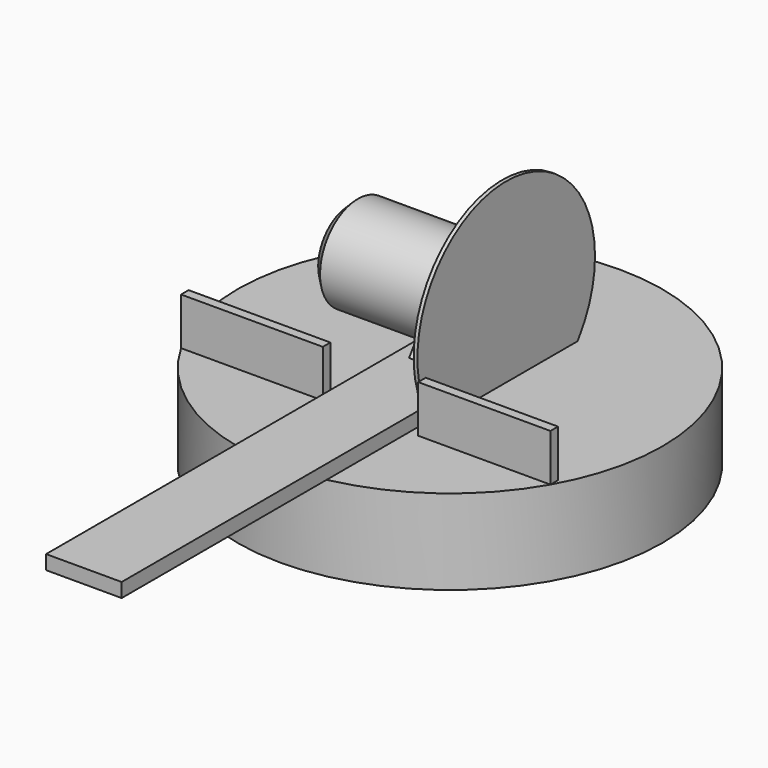
from build123d import *

# Parameters (mm, degrees)
F0_W          = 80
F0_H          = 600
F1_DEPTH      = 15
F3_DEPTH      = 43
F3_DEPTH_BACK = 120
F4_DEPTH      = 25
F4_DEPTH_BACK = 25
F5_R          = 117.5
F6_DEPTH      = 4
F8_W          = 25
F8_H          = 90
F10_R         = 30
F11_SIZE      = 10
F13_DEPTH     = 72.001
F14_T1_DEPTH  = 30
F14_T4_ANGLE  = 90
F14_T8_DEPTH  = 72.5
F14_S9_R      = 50
F14_T10_DEPTH = 38
F14_T14_DEPTH = 72.5
F14_S15_R     = 50
F14_T16_DEPTH = 38
F14_T18_ANGLE = 90
F14_T22_DEPTH = 67.4896230895
F14_T25_ANGLE = 180
F14_T27_ANGLE = 180
F14_T29_ANGLE = 90
F14_T31_ANGLE = 90
F14_T35_DEPTH = 67.4896230895
F14_T38_ANGLE = 180
F14_T40_ANGLE = 180
F15_R         = 225
F16_DEPTH     = 90
F17_W         = 140
F17_H         = 10
F17_W_2       = 150
F18_DEPTH     = 50


# Not quite as in the source:
# - a fillet or chamfer that OpenCascade refuses, or shapes differently, is made with other operations: its cross-section is extruded or revolved along the edge and cut away or added


with BuildPart() as f1:
    # F0 (on Top) → F1 (new body)
    with BuildSketch(Plane.XY):
        with Locations((0, -200)):
            Rectangle(F0_W, F0_H)
    extrude(amount=-F1_DEPTH)


with BuildPart() as f3:
    # F2 (on Right) → F3 (new body, two sides)
    with BuildSketch(Plane.YZ) as f3_sk:
        with BuildLine():
            Line((0, 55), (-28.6788218176, 14.0423977856))
            ThreePointArc((-28.6788218176, 14.0423977855), (0, 5), (28.6788218176, 14.0423977855))
            Line((28.6788218176, 14.0423977856), (0, 55))
        make_face()
        with BuildLine():
            ThreePointArc((28.6788218176, 14.0423977855), (44.3505416589, 31.9125693382), (50, 55))
            ThreePointArc((50, 55), (-23.0874306618, 99.3505416589), (-28.6788218176, 14.0423977855))
            Line((-28.6788218176, 14.0423977856), (0, 55))
            Line((0, 55), (28.6788218176, 14.0423977856))
        make_face()
    extrude(amount=F3_DEPTH)
    extrude(f3_sk.sketch, amount=-F3_DEPTH_BACK)

    # F2 (on Right) → F4 (join, two sides)
    with BuildSketch(Plane.YZ) as f4_sk:
        with BuildLine():
            ThreePointArc((28.6788218176, 14.0423977855), (0, 5), (-28.6788218176, 14.0423977855))
            Line((-28.6788218176, 14.0423977856), (-49.0145276747, -15))
            Line((-49.0145276747, -15), (49.0145276747, -15))
            Line((49.0145276747, -15), (28.6788218176, 14.0423977856))
        make_face()
    extrude(amount=F4_DEPTH)
    extrude(f4_sk.sketch, amount=-F4_DEPTH_BACK)

    # F8 (on offset) → F9 (join, up to the next surface of F3)
    with BuildSketch(Plane.XZ.offset(-120)):
        with Locations((-12.5, 50)):
            Rectangle(F8_W, F8_H)
    extrude(until=Until.NEXT)

    # F10
    f10_edges = [f3.edges().sort_by_distance(p)[0] for p in [
        (-12.5, 120, 95),
        (-12.5, 120, 5),
    ]]
    fillet(f10_edges, radius=F10_R)

    # F11
    f11_edges = [f3.edges().sort_by_distance(p)[0] for p in [
        (-120, 28.678822, 95.957602),
    ]]
    chamfer(f11_edges, length=F11_SIZE)

    # F12 (on face) → F13 (cut, through all)
    with BuildSketch(Plane(origin=(-25, 0, 0), x_dir=(0, -1, 0), z_dir=(-1, 0, 0))):
        with BuildLine():
            Line((-75, 35), (-75, 65))
            ThreePointArc((-75, 65), (-90, 80), (-105, 65))
            Line((-105, 65), (-105, 35))
            ThreePointArc((-105, 35), (-90, 20), (-75, 35))
        make_face()
    extrude(amount=-F13_DEPTH, mode=Mode.SUBTRACT)

    # F14: fillet of radius 5 on 18 edges, made by hand

    # F14_s2 → F14_t1 (cut)
    with BuildSketch(Plane.XY.offset(35)):
        with BuildLine():
            ThreePointArc((-25, 110), (-23.5355339059, 106.4644660941), (-20, 105))
            Line((-20, 105), (-25, 105))
            Line((-25, 105), (-25, 110))
        make_face()
        with BuildLine():
            ThreePointArc((0, 115), (-1.4644660941, 118.5355339059), (-5, 120))
            Line((-5, 120), (0, 120))
            Line((0, 120), (0, 115))
        make_face()
        with BuildLine():
            ThreePointArc((0, 110), (-1.4644660941, 106.4644660941), (-5, 105))
            Line((-5, 105), (0, 105))
            Line((0, 105), (0, 110))
        make_face()
        with BuildLine():
            ThreePointArc((-25, 115), (-23.5355339059, 118.5355339059), (-20, 120))
            Line((-20, 120), (-25, 120))
            Line((-25, 120), (-25, 115))
        make_face()
        with BuildLine():
            ThreePointArc((-25, 70), (-23.5355339059, 73.5355339059), (-20, 75))
            Line((-20, 75), (-25, 75))
            Line((-25, 75), (-25, 70))
        make_face()
        with BuildLine():
            ThreePointArc((0, 70), (-1.4644660941, 73.5355339059), (-5, 75))
            Line((-5, 75), (0, 75))
            Line((0, 75), (0, 70))
        make_face()
    extrude(amount=F14_T1_DEPTH, mode=Mode.SUBTRACT)

    # F14_s3 → F14_t4 (revolve, cut)
    with BuildSketch(Plane.XY.offset(65)):
        with BuildLine():
            ThreePointArc((-25, 115), (-23.5355339059, 118.5355339059), (-20, 120))
            Line((-20, 120), (-25, 120))
            Line((-25, 120), (-25, 115))
        make_face()
    revolve(axis=Axis((-25, 90, 65), (1, 0, 0)), revolution_arc=F14_T4_ANGLE, mode=Mode.SUBTRACT)


with BuildPart() as f6:
    # F5 (on face) → F6 (new body)
    with BuildSketch(Plane.YZ.offset(43)):
        with Locations((0, 55)):
            Circle(F5_R)
    extrude(amount=F6_DEPTH)


with BuildPart() as f14_tool6:
    # F14_s7 → F14_t8 (new body)
    with BuildSketch(Plane.XZ.offset(-90)):
        with BuildLine():
            ThreePointArc((-20, 95), (-23.5355339059, 93.5355339059), (-25, 90))
            Line((-25, 90), (-25, 95))
            Line((-25, 95), (-20, 95))
        make_face()
    extrude(amount=F14_T8_DEPTH)

    # F14_s9 → F14_t10 (cut, symmetric)
    with BuildSketch(Plane.YZ.offset(-22.5)):
        with Locations((0, 55)):
            Circle(F14_S9_R)
    extrude(amount=F14_T10_DEPTH, both=True, mode=Mode.SUBTRACT)


with BuildPart() as f3_1:
    add(f3.part)

    # F14_t5: cut F14_tool6
    add(f14_tool6.part, mode=Mode.SUBTRACT)


with BuildPart() as f14_tool12:
    # F14_s13 → F14_t14 (new body)
    with BuildSketch(Plane.XZ.offset(-90)):
        with BuildLine():
            ThreePointArc((-5, 95), (-1.4644660941, 93.5355339059), (0, 90))
            Line((0, 90), (0, 95))
            Line((0, 95), (-5, 95))
        make_face()
    extrude(amount=F14_T14_DEPTH)

    # F14_s15 → F14_t16 (cut, symmetric)
    with BuildSketch(Plane.YZ.offset(-2.5)):
        with Locations((0, 55)):
            Circle(F14_S15_R)
    extrude(amount=F14_T16_DEPTH, both=True, mode=Mode.SUBTRACT)


with BuildPart() as f3_2:
    add(f3_1.part)

    # F14_t11: cut F14_tool12
    add(f14_tool12.part, mode=Mode.SUBTRACT)

    # F14_s17 → F14_t18 (revolve, cut)
    with BuildSketch(Plane.XZ.offset(-90)):
        with BuildLine():
            ThreePointArc((-25, 10), (-23.5355339059, 6.4644660941), (-20, 5))
            Line((-20, 5), (-25, 5))
            Line((-25, 5), (-25, 10))
        make_face()
    revolve(axis=Axis((-25, 90, 35), (1, 0, 0)), revolution_arc=F14_T18_ANGLE, mode=Mode.SUBTRACT)


with BuildPart() as f14_tool20:
    # F14_s21 → F14_t22 (new body)
    with BuildSketch(Plane.XZ.offset(-90)):
        with BuildLine():
            ThreePointArc((-25, 10), (-23.5355339059, 6.4644660941), (-20, 5))
            Line((-20, 5), (-25, 5))
            Line((-25, 5), (-25, 10))
        make_face()
    extrude(amount=F14_T22_DEPTH)

    split(bisect_by=Plane(origin=(0, 25.8415470716, 18.0944460585), x_dir=(1, 0, 0), z_dir=(0, 0.8191520443, 0.5735764364)), keep=Keep.TOP)


with BuildPart() as f3_3:
    add(f3_2.part)

    # F14_t19: cut F14_tool20
    add(f14_tool20.part, mode=Mode.SUBTRACT)

    # F14_s24 → F14_t25 (revolve, cut)
    with BuildSketch(Plane.XY.offset(65)):
        with BuildLine():
            ThreePointArc((-25, 70), (-23.5355339059, 73.5355339059), (-20, 75))
            Line((-20, 75), (-25, 75))
            Line((-25, 75), (-25, 70))
        make_face()
    revolve(axis=Axis((-25, 90, 65), (-1, 0, 0)), revolution_arc=F14_T25_ANGLE, mode=Mode.SUBTRACT)

    # F14_s26 → F14_t27 (revolve, cut)
    with BuildSketch(Plane.XY.offset(35)):
        with BuildLine():
            ThreePointArc((-25, 110), (-23.5355339059, 106.4644660941), (-20, 105))
            Line((-20, 105), (-25, 105))
            Line((-25, 105), (-25, 110))
        make_face()
    revolve(axis=Axis((-25, 90, 35), (-1, 0, 0)), revolution_arc=F14_T27_ANGLE, mode=Mode.SUBTRACT)

    # F14_s28 → F14_t29 (revolve, cut)
    with BuildSketch(Plane.XZ.offset(-90)):
        with BuildLine():
            ThreePointArc((0, 10), (-1.4644660941, 6.4644660941), (-5, 5))
            Line((-5, 5), (0, 5))
            Line((0, 5), (0, 10))
        make_face()
    revolve(axis=Axis((0, 90, 35), (1, 0, 0)), revolution_arc=F14_T29_ANGLE, mode=Mode.SUBTRACT)

    # F14_s30 → F14_t31 (revolve, cut)
    with BuildSketch(Plane.XY.offset(65)):
        with BuildLine():
            ThreePointArc((0, 115), (-1.4644660941, 118.5355339059), (-5, 120))
            Line((-5, 120), (0, 120))
            Line((0, 120), (0, 115))
        make_face()
    revolve(axis=Axis((0, 90, 65), (1, 0, 0)), revolution_arc=F14_T31_ANGLE, mode=Mode.SUBTRACT)


with BuildPart() as f14_tool33:
    # F14_s34 → F14_t35 (new body)
    with BuildSketch(Plane.XZ.offset(-90)):
        with BuildLine():
            ThreePointArc((0, 10), (-1.4644660941, 6.4644660941), (-5, 5))
            Line((-5, 5), (0, 5))
            Line((0, 5), (0, 10))
        make_face()
    extrude(amount=F14_T35_DEPTH)

    split(bisect_by=Plane(origin=(0, 25.8415470716, 18.0944460585), x_dir=(1, 0, 0), z_dir=(0, 0.8191520443, 0.5735764364)), keep=Keep.TOP)


with BuildPart() as f3_4:
    add(f3_3.part)

    # F14_t32: cut F14_tool33
    add(f14_tool33.part, mode=Mode.SUBTRACT)

    # F14_s37 → F14_t38 (revolve, cut)
    with BuildSketch(Plane.XY.offset(35)):
        with BuildLine():
            ThreePointArc((0, 110), (-1.4644660941, 106.4644660941), (-5, 105))
            Line((-5, 105), (0, 105))
            Line((0, 105), (0, 110))
        make_face()
    revolve(axis=Axis((0, 90, 35), (-1, 0, 0)), revolution_arc=F14_T38_ANGLE, mode=Mode.SUBTRACT)

    # F14_s39 → F14_t40 (revolve, cut)
    with BuildSketch(Plane.XY.offset(65)):
        with BuildLine():
            ThreePointArc((0, 70), (-1.4644660941, 73.5355339059), (-5, 75))
            Line((-5, 75), (0, 75))
            Line((0, 75), (0, 70))
        make_face()
    revolve(axis=Axis((0, 90, 65), (-1, 0, 0)), revolution_arc=F14_T40_ANGLE, mode=Mode.SUBTRACT)


with BuildPart() as f16:
    # F15 (on face) → F16 (new body)
    with BuildSketch(Plane(origin=(0, 0, -15), x_dir=(1, 0, 0), z_dir=(0, 0, -1))):
        with Locations((-5.6465086527, 8.5678258911)):
            Circle(F15_R)
    extrude(amount=F16_DEPTH)

    # F17 (on face) → F18 (join)
    with BuildSketch(Plane.XY.offset(-15)):
        with Locations((119.8218278454, -115)):
            Rectangle(F17_W, F17_H)
        with Locations((-126.1148451509, -115)):
            Rectangle(F17_W_2, F17_H)
    extrude(amount=F18_DEPTH)


solid = Compound([f1.part, f6.part, f3_4.part, f16.part])
